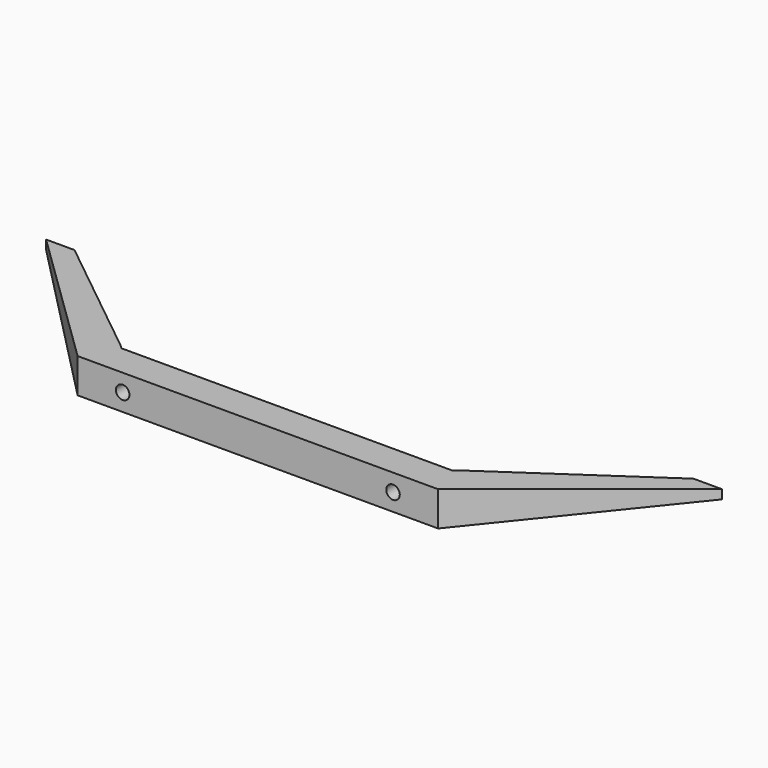
from build123d import *

# Parameters (mm, degrees)
F1_DEPTH    = 8
F2_R        = 1.5
F3_DEPTH    = 8
F4_DEPTH    = 2
F5_SIZE2    = 5
F5_SIZE     = 37
F6_T1_DEPTH = 198.6904330104


# Not quite as in the source:
# - a fillet or chamfer that OpenCascade refuses, or shapes differently, is made with other operations: its cross-section is extruded or revolved along the edge and cut away or added


with BuildPart() as f1:
    # F0 (on Top) → F1 (new body)
    with BuildSketch(Plane.XY):
        Polygon((0, -4), (40, -4), (75, 31), (63.686291501, 31), (36.686291501, 4), (0, 4), align=None)
    extrude(amount=F1_DEPTH)

    # F2 (on face) → F3 (cut, through all)
    with BuildSketch(Plane(origin=(0, 4, 0), x_dir=(-1, 0, 0), z_dir=(0, 1, 0))):
        with Locations((-30, 4)):
            Circle(F2_R)
    extrude(amount=-F3_DEPTH, mode=Mode.SUBTRACT)

    # F2 (on face) → F4 (cut)
    with BuildSketch(Plane(origin=(0, 4, 0), x_dir=(-1, 0, 0), z_dir=(0, 1, 0))):
        Polygon((-28.4122867597, 1.25), (-26.8245735195, 4), (-28.4122867597, 6.75), (-31.5877132403, 6.75), (-33.1754264805, 4), (-31.5877132403, 1.25), align=None)
        with Locations((-30, 4)):
            Circle(F2_R, mode=Mode.SUBTRACT)
    extrude(amount=-F4_DEPTH, mode=Mode.SUBTRACT)

    # F5
    f5_edges = [f1.edges().sort_by_distance(p)[0] for p in [
        (63.686292, 31, 4),
    ]]
    f5_side = f1.faces().sort_by_distance((50.186292, 17.5, 4))[0]
    chamfer(f5_edges, length=F5_SIZE, length2=F5_SIZE2, reference=f5_side)

    # F6: chamfer of 37 x 3 on 2 edges, made by hand

    # F6_s2 → F6_t1 (cut)
    with BuildSketch(Plane.YZ.offset(-27.5020707547)):
        Polygon((-6, 0), (31, 3), (31, 0), align=None)
        Polygon((31, 5), (-6, 8), (31, 8), align=None)
    extrude(amount=F6_T1_DEPTH, mode=Mode.SUBTRACT)

    # F7: F1 across plane


with BuildPart() as f1_1:
    add(f1.part)
    add(f1.part.mirror(Plane.YZ))


solid = f1_1.part
